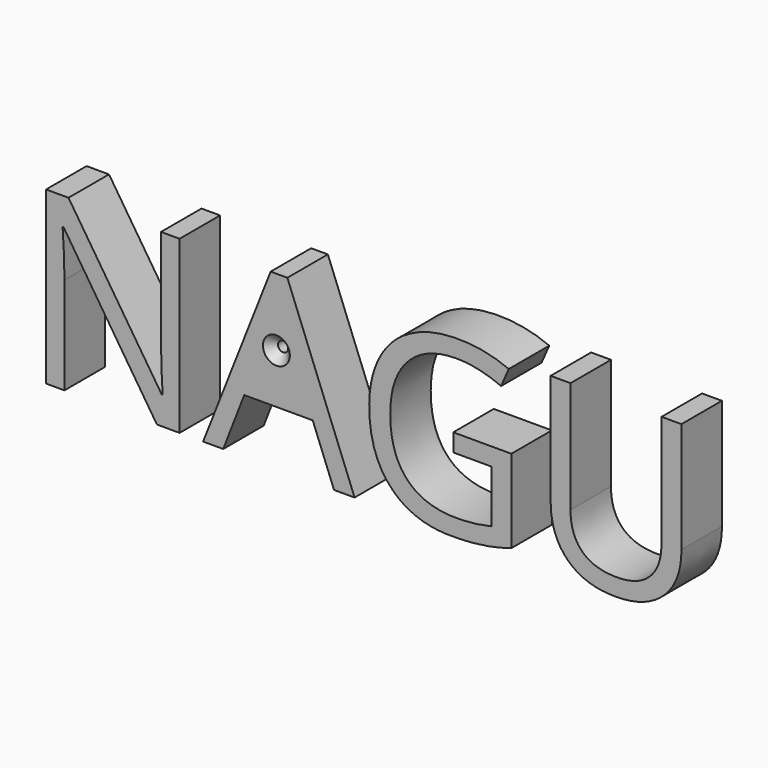
from build123d import *

# Parameters (mm, degrees)
F0_TEXT_SIZE   = 120.1337203383
F1_DEPTH       = 25.4
F4_D           = 5.1054
F4_DEPTH       = 16.51
F4_CSINK_D     = 13.4874
F4_CSINK_ANGLE = 90
F4_TIP         = 1.5338169022


# Not quite as in the source:
# - Text() gives the source's letters only with a copy of the font that has no kerning and outlines rounded to 1/6400 em; it was checked with that copy


with BuildPart() as f1:
    # F0 (on Front) → F1 (new body)
    with BuildSketch(Plane.XZ):
        with Locations((-75.998865068, 0)):
            Text('NAGU', F0_TEXT_SIZE, font='Open Sans', text_align=(TextAlign.LEFT, TextAlign.BOTTOM))
        with BuildLine():
            Line((38.747608749, 36.2465959333), (66.4909897896, 36.2465959333))
            Line((66.4909897896, 36.2465959333), (56.5048742865, 62.8261815582))
            add(Edge.make_bspline(
                [(56.5048742865, 62.8261815582), (54.5714722248, 67.8755519912), (52.5254448003, 75.1962005743)],
                knots=[0, 0, 0, 1, 1, 1], degree=2))
            add(Edge.make_bspline(
                [(52.5254448003, 75.1962005743), (51.2302531279, 69.5649324334), (48.8275787211, 62.8261815582)],
                knots=[0, 0, 0, 1, 1, 1], degree=2))
            Line((48.8275787211, 62.8261815582), (38.747608749, 36.2465959333))
        make_face()
    extrude(amount=F1_DEPTH)

    # F4
    with Locations(Plane.XZ.offset(25.4)):
        with Locations((51.3530559838, 52.2268228233)):
            CounterSinkHole(F4_D / 2, F4_CSINK_D / 2, depth=F4_DEPTH, counter_sink_angle=F4_CSINK_ANGLE)
            with Locations((0, 0, -(F4_DEPTH + F4_TIP / 2))):  # 118° drill point
                Cone(0, F4_D / 2, F4_TIP, mode=Mode.SUBTRACT)


solid = f1.part
